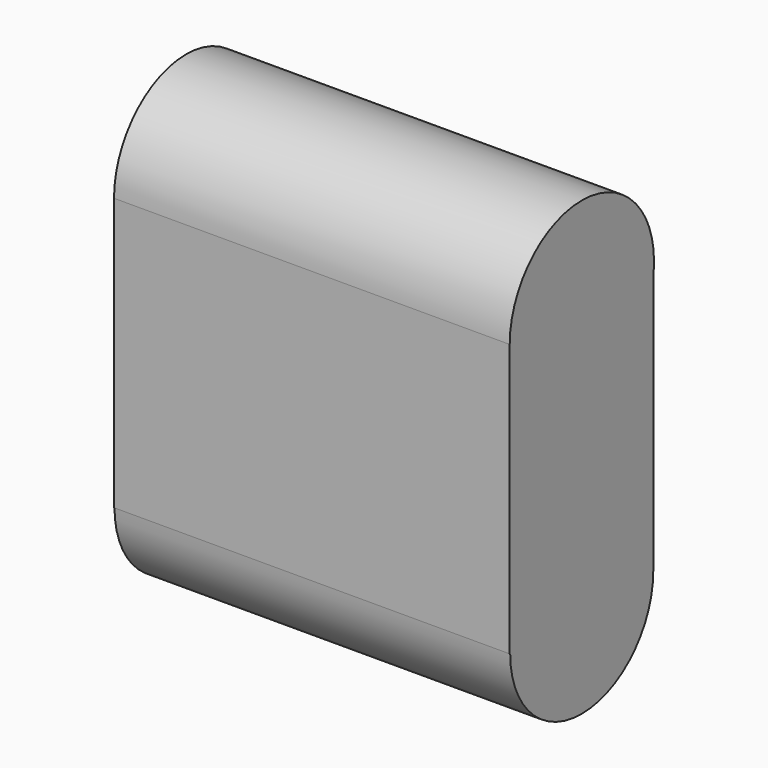
from build123d import *

# Parameters (mm, degrees)
F3_DEPTH = 25


# Not quite as in the source:
# - the program builds the solid bodies; features that only make, move or delete a surface that nothing else refers to are left out


with BuildPart() as f3:
    # F2 (on Right) → F3 (new body)
    with BuildSketch(Plane.YZ):
        with BuildLine():
            ThreePointArc((-56.4248897135, 62.7899920644), (-56.4100056303, 63.0273500708), (-56.4050413852, 63.2651224732))
            ThreePointArc((-56.4050413852, 63.2651224732), (-62.1018148959, 68.9618959839), (-67.7985884065, 63.2651224732))
            Line((-67.7985884065, 63.2651224732), (-56.4248897135, 63.2651224732))
            Line((-56.4248897135, 63.2651224732), (-56.4248897135, 62.7899920644))
        make_face()
        with BuildLine():
            Line((-56.4628131563, 46.0544750094), (-67.7606649638, 46.0544750094))
            ThreePointArc((-67.7606649638, 46.0544750094), (-62.11173906, 40.4055491057), (-56.4628131563, 46.0544750094))
        make_face()
        with BuildLine():
            Line((-56.4248897135, 63.2651224732), (-67.7985884065, 63.2651224732))
            ThreePointArc((-67.7985884065, 63.2651224732), (-62.3395872983, 57.5733132076), (-56.4248897135, 62.7899920644))
            Line((-56.4248897135, 62.7899920644), (-56.4248897135, 63.2651224732))
        make_face()
        with BuildLine():
            ThreePointArc((-56.4248897135, 62.7899920644), (-62.3395872983, 57.5733132076), (-67.7985884065, 63.2651224732))
            Line((-67.7985884065, 63.2651224732), (-67.7985884065, 46.0544750094))
            Line((-67.7985884065, 46.0544750094), (-67.7606649638, 46.0544750094))
            ThreePointArc((-67.7606649638, 46.0544750094), (-62.11173906, 51.7034009132), (-56.4628131563, 46.0544750094))
            Line((-56.4628131563, 46.0544750094), (-56.4248897135, 46.0544750094))
            Line((-56.4248897135, 46.0544750094), (-56.4248897135, 62.7899920644))
        make_face()
        with BuildLine():
            ThreePointArc((-56.4628131563, 46.0544750094), (-62.11173906, 51.7034009132), (-67.7606649638, 46.0544750094))
            Line((-67.7606649638, 46.0544750094), (-56.4628131563, 46.0544750094))
        make_face()
    extrude(amount=F3_DEPTH)


solid = f3.part
